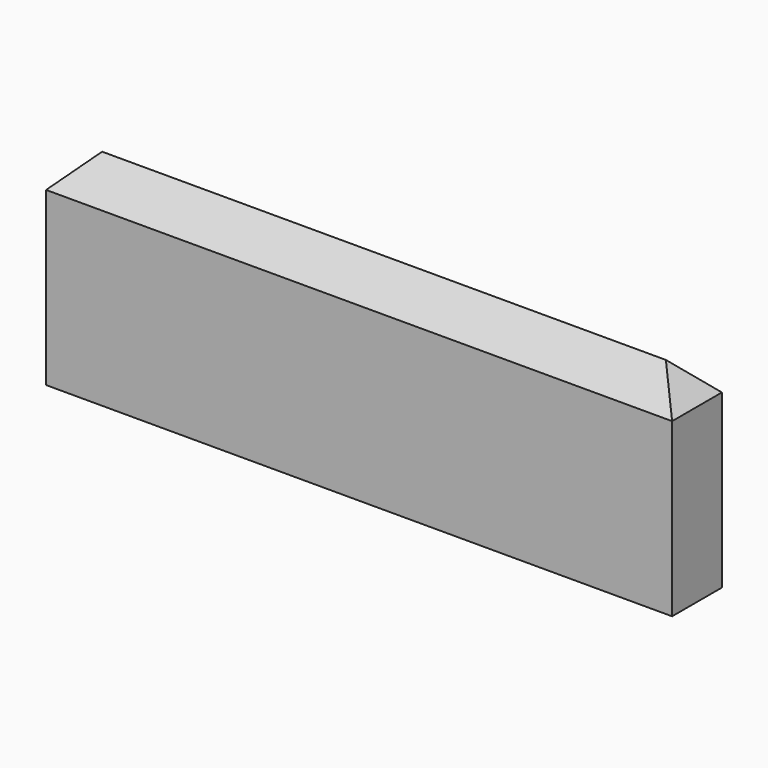
from build123d import *

# Parameters (mm, degrees)
F0_W          = 91.08898
F0_H          = 9.059988
F1_DEPTH      = 15
F1_TAPER      = 45
F1_DEPTH_BACK = 25


with BuildPart() as f1:
    # F0 (on Top) → F1 (new body, two sides)
    with BuildSketch(Plane.XY) as f1_sk:
        with Locations((1.610279, 41.666087)):
            Rectangle(F0_W, F0_H)
    extrude(amount=F1_DEPTH, taper=F1_TAPER)
    extrude(f1_sk.sketch, amount=-F1_DEPTH_BACK)


solid = f1.part
